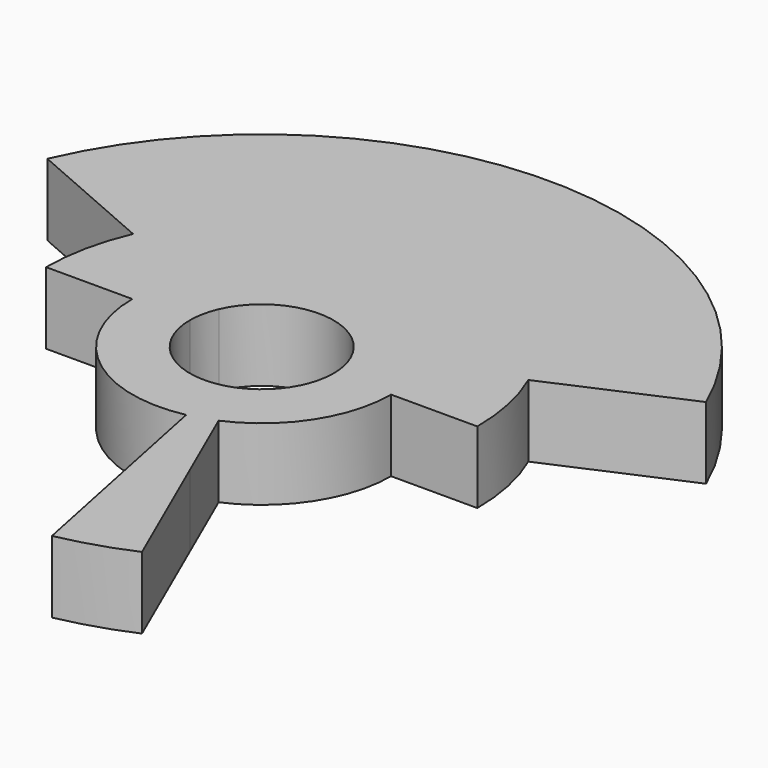
from build123d import *

# Parameters (mm, degrees)
F1_DEPTH = 2.54


with BuildPart() as f1:
    # F0 (on Top) → F1 (new body)
    with BuildSketch(Plane.XY):
        with BuildLine():
            ThreePointArc((2.327948453, 1.016), (2.4864220348, 0.518946495), (2.54, 0))
            Line((2.54, 0), (4.572, 0))
            ThreePointArc((4.572, 0), (4.4755596627, 0.9341036909), (4.1903072155, 1.8288))
            Line((4.1903072155, 1.8288), (2.327948453, 1.016))
        make_face()
        with BuildLine():
            Line((4.572, 0), (2.54, 0))
            ThreePointArc((2.54, 0), (2.1251164674, -1.3912152961), (1.016, -2.327948453))
            Line((1.016, -2.327948453), (1.8288, -4.1903072155))
            ThreePointArc((1.8288, -4.1903072155), (3.8252096413, -2.5041875329), (4.572, 0))
        make_face()
        with BuildLine():
            ThreePointArc((-2.327948453, 1.016), (0, 2.54), (2.327948453, 1.016))
            Line((2.327948453, 1.016), (4.1903072155, 1.8288))
            ThreePointArc((4.1903072155, 1.8288), (0, 4.572), (-4.1903072155, 1.8288))
            Line((-4.1903072155, 1.8288), (-2.327948453, 1.016))
        make_face()
        with BuildLine():
            ThreePointArc((-2.54, 0), (-2.4864220348, 0.518946495), (-2.327948453, 1.016))
            Line((-2.327948453, 1.016), (-4.1903072155, 1.8288))
            ThreePointArc((-4.1903072155, 1.8288), (-4.4755596627, 0.9341036909), (-4.572, 0))
            Line((-4.572, 0), (-2.54, 0))
        make_face()
        with BuildLine():
            Line((0.9144, -4.4796268416), (0.508, -2.4886815787))
            ThreePointArc((0.508, -2.4886815787), (-1.6064370514, -1.9674755399), (-2.54, 0))
            Line((-2.54, 0), (-4.572, 0))
            ThreePointArc((-4.572, 0), (-2.8915866925, -3.5414559718), (0.9144, -4.4796268416))
        make_face()
        with BuildLine():
            ThreePointArc((1.016, -2.327948453), (0.7662263272, -2.4216724005), (0.508, -2.4886815787))
            Line((0.508, -2.4886815787), (0.9144, -4.4796268416))
            ThreePointArc((0.9144, -4.4796268416), (1.3792073889, -4.359010321), (1.8288, -4.1903072155))
            Line((1.8288, -4.1903072155), (1.016, -2.327948453))
        make_face()
        with BuildLine():
            ThreePointArc((4.1903072155, 1.8288), (4.4755596627, 0.9341036909), (4.572, 0))
            Line((4.572, 0), (7.62, 0))
            ThreePointArc((7.62, 0), (7.4592661045, 1.5568394849), (6.9838453591, 3.048))
            Line((6.9838453591, 3.048), (4.1903072155, 1.8288))
        make_face()
        with BuildLine():
            ThreePointArc((-4.1903072155, 1.8288), (0, 4.572), (4.1903072155, 1.8288))
            Line((4.1903072155, 1.8288), (6.9838453591, 3.048))
            ThreePointArc((6.9838453591, 3.048), (0, 7.62), (-6.9838453591, 3.048))
            Line((-6.9838453591, 3.048), (-4.1903072155, 1.8288))
        make_face()
        with BuildLine():
            ThreePointArc((-4.572, 0), (-4.4755596627, 0.9341036909), (-4.1903072155, 1.8288))
            Line((-4.1903072155, 1.8288), (-6.9838453591, 3.048))
            ThreePointArc((-6.9838453591, 3.048), (-7.4592661045, 1.5568394849), (-7.62, 0))
            Line((-7.62, 0), (-4.572, 0))
        make_face()
        with BuildLine():
            ThreePointArc((1.8288, -4.1903072155), (1.3792073889, -4.359010321), (0.9144, -4.4796268416))
            Line((0.9144, -4.4796268416), (1.524, -7.466044736))
            ThreePointArc((1.524, -7.466044736), (2.2986789815, -7.2650172016), (3.048, -6.9838453591))
            Line((3.048, -6.9838453591), (1.8288, -4.1903072155))
        make_face()
        with BuildLine():
            ThreePointArc((-6.9838453591, 3.048), (0, 7.62), (6.9838453591, 3.048))
            Line((6.9838453591, 3.048), (11.6397422652, 5.08))
            ThreePointArc((11.6397422652, 5.08), (0, 12.7), (-11.6397422652, 5.08))
            Line((-11.6397422652, 5.08), (-6.9838453591, 3.048))
        make_face()
        with BuildLine():
            ThreePointArc((3.048, -6.9838453591), (2.2986789815, -7.2650172016), (1.524, -7.466044736))
            Line((1.524, -7.466044736), (2.54, -12.4434078933))
            ThreePointArc((2.54, -12.4434078933), (3.8311316358, -12.1083620027), (5.08, -11.6397422652))
            Line((5.08, -11.6397422652), (3.048, -6.9838453591))
        make_face()
    extrude(amount=F1_DEPTH)


solid = f1.part
